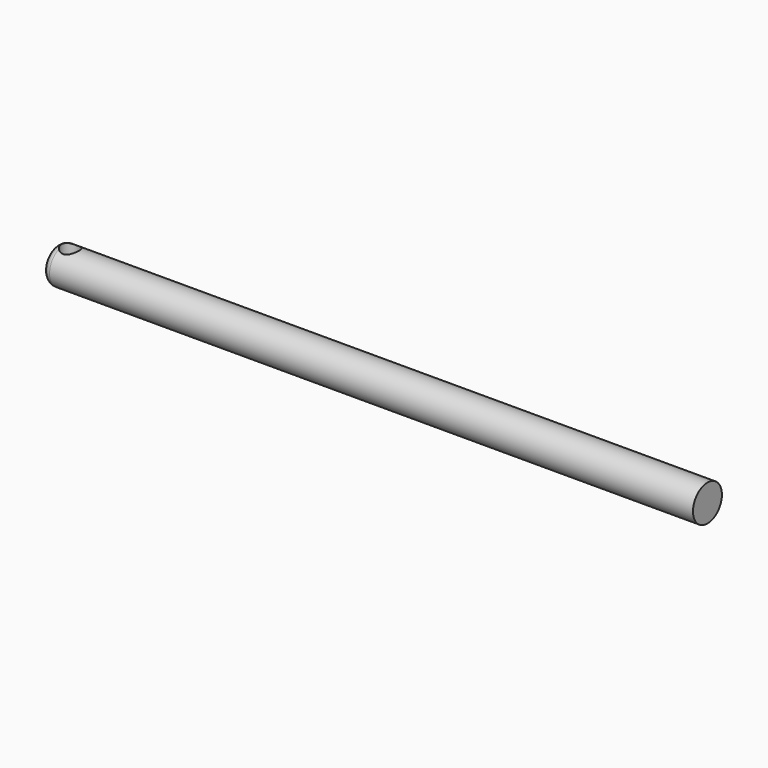
from build123d import *

# Parameters (mm, degrees)
F0_R     = 12.7
F1_DEPTH = 457.2
F2_R     = 6.35
F3_DEPTH = 12.7


# Not quite as in the source:
# - a fillet or chamfer that OpenCascade refuses, or shapes differently, is made with other operations: its cross-section is extruded or revolved along the edge and cut away or added


with BuildPart() as f1:
    # F0 (on Right) → F1 (new body)
    with BuildSketch(Plane.YZ):
        Circle(F0_R)
    extrude(amount=F1_DEPTH)

    # F2 (on Top) → F3 (cut, symmetric)
    with BuildSketch(Plane.XY):
        with Locations((9.525, 0)):
            Circle(F2_R)
    extrude(amount=F3_DEPTH, both=True, mode=Mode.SUBTRACT)

    # F4: fillet of radius 5.08 on 1 edges, made by hand

    # F4_s1 → F4_t2 (revolve, cut)
    with BuildSketch(Plane.XY):
        with BuildLine():
            ThreePointArc((5.08, 12.7), (1.4878975516, 11.2121024484), (0, 7.62))
            Line((0, 7.62), (0, 12.7))
            Line((0, 12.7), (5.08, 12.7))
        make_face()
    revolve(axis=Axis((0, 0, 0), (1, 0, 0)), mode=Mode.SUBTRACT)


solid = f1.part
